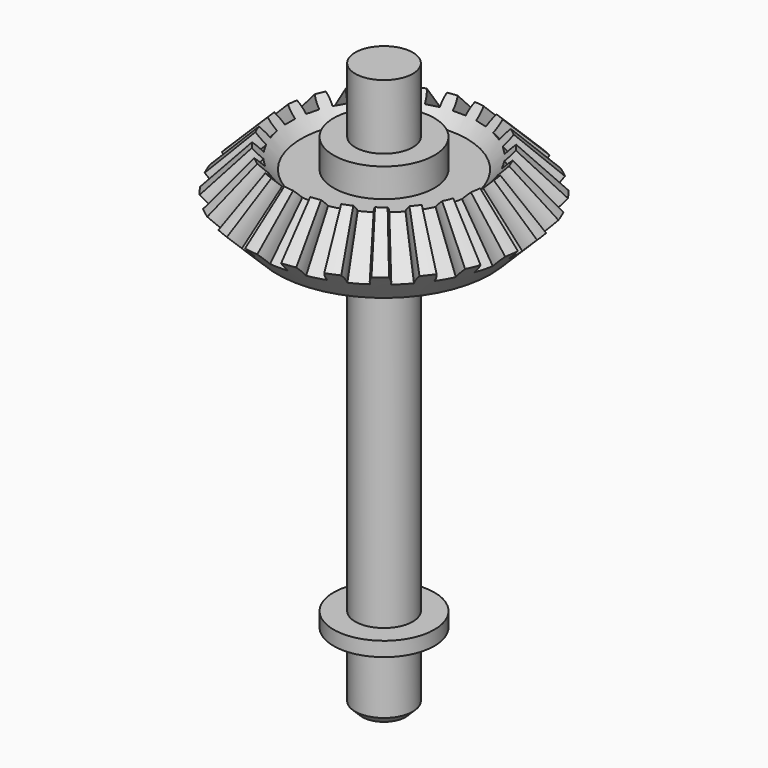
from build123d import *

# Parameters (mm, degrees)
F6_COPIES_COUNT = 24
F9_SIZE         = 1


# Not quite as in the source:
# - a pattern or mirror of a feature is missing from the dataset's text; its kind, count and spacing are read off the source's solid


with BuildPart() as f2:
    # F1 (on Front) → F2 (revolve)
    with BuildSketch(Plane.XZ):
        Polygon((0, 8), (0, 0), (14.8284271247, 0), (20, 5.1715728753), (14.3431457505, 10.8284271247), (11.5147186258, 8), align=None)
    revolve(axis=Axis((0, 0, 0), (0, 0, -1)))

    # F4 (on line) → F6 section 0
    with BuildSketch(Plane(origin=(7.4142135624, 0, -7.4142135624), x_dir=(0.7071067812, 0, 0.7071067812), z_dir=(0.7071067812, 0, -0.7071067812)), mode=Mode.PRIVATE) as f6_s0:
        with BuildLine():
            ThreePointArc((20.2989898732, 3.1598300563), (17.9751555465, 1.7437073078), (15.2989898732, 1.25))
            Line((15.2989898732, 1.25), (15.2989898732, -1.25))
            ThreePointArc((15.2989898732, -1.25), (17.9751555465, -1.7437073078), (20.2989898732, -3.1598300563))
            Line((20.2989898732, -3.1598300563), (20.2989898732, 3.1598300563))
        make_face()
    f6 = loft([f6_s0.sketch, Vertex(0, 0, 25.1715728753)], mode=Mode.SUBTRACT)

    # F6_copies: F6 ×24 about axis
    f6_copies_axis = Axis((0, 0, 0), (0, 0, 1))
    for i in range(1, F6_COPIES_COUNT):
        add(f6.rotate(f6_copies_axis, i * 360 / F6_COPIES_COUNT), mode=Mode.SUBTRACT)

    # F7 (on Front) → F8 (revolve)
    with BuildSketch(Plane.XZ):
        Polygon((7, 12), (4, 12), (4, 21), (0, 21), (0, -58), (4, -58), (4, -48), (7, -48), (7, -46), (4, -46), (4, -2), (7, -2), align=None)
    revolve(axis=Axis((0, 0, 0), (0, 0, -1)))

    # F9
    f9_edges = [f2.edges().sort_by_distance(p)[0] for p in [
        (-4, 0, -58),
    ]]
    chamfer(f9_edges, length=F9_SIZE)


solid = f2.part
